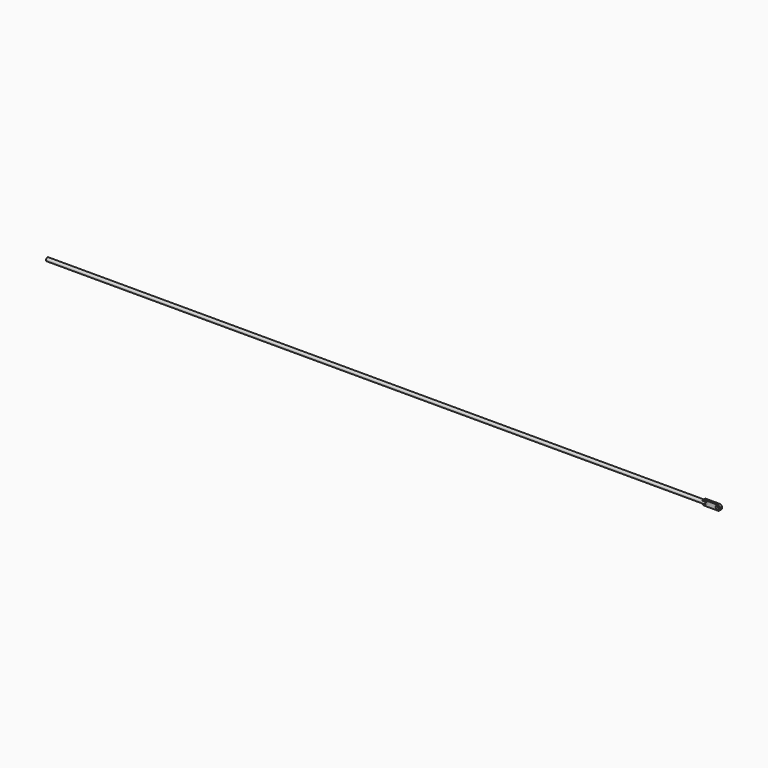
from build123d import *

# Parameters (mm, degrees)
F0_R         = 1.5875
F1_DEPTH     = 304.8
F3_DEPTH     = 1.0795
F4_T4_DEPTH  = 15.027948453
F4_S5_R      = 1.5875
F4_T6_DEPTH  = 9
F4_T10_DEPTH = 15.027948453
F4_S11_R     = 1.5875
F4_T12_DEPTH = 9
F5_R         = 1.5875
F6_DEPTH     = 2.6680001


# Not quite as in the source:
# - a fillet or chamfer that OpenCascade refuses, or shapes differently, is made with other operations: its cross-section is extruded or revolved along the edge and cut away or added


with BuildPart() as f1:
    # F0 (on Right) → F1 (new body, symmetric)
    with BuildSketch(Plane.YZ):
        Circle(F0_R)
    extrude(amount=F1_DEPTH, both=True)

    # F2 (on Front) → F3 (join, symmetric)
    with BuildSketch(Plane.XZ):
        with BuildLine():
            Line((304.7385620117, -2.3473887456), (317.4385620117, -2.3473887456))
            ThreePointArc((317.4385620117, -2.3473887456), (318.7856004299, -1.7894271638), (319.3435620117, -0.4423887456))
            Line((319.3435620117, -0.4423887456), (319.3435620117, 0.4423887456))
            ThreePointArc((319.3435620117, 0.4423887456), (318.7856004299, 1.7894271638), (317.4385620117, 2.3473887456))
            Line((317.4385620117, 2.3473887456), (304.7385620117, 2.3473887456))
            ThreePointArc((304.7385620117, 2.3473887456), (303.3915235936, 1.7894271638), (302.8335620117, 0.4423887456))
            Line((302.8335620117, 0.4423887456), (302.8335620117, -0.4423887456))
            ThreePointArc((302.8335620117, -0.4423887456), (303.3915235936, -1.7894271638), (304.7385620117, -2.3473887456))
        make_face()
    extrude(amount=F3_DEPTH, both=True)

    # F4: fillet of radius 2.54 on 2 edges, made by hand


with BuildPart() as f4_tool2:
    # F4_s3 → F4_t4 (new body)
    with BuildSketch(Plane.XY.offset(7.5139742265)):
        with BuildLine():
            ThreePointArc((307.34, -1.0795), (305.5439487758, -1.8234487758), (304.8, -3.6195))
            Line((304.8, -3.6195), (304.8, -1.0795))
            Line((304.8, -1.0795), (307.34, -1.0795))
        make_face()
    extrude(amount=-F4_T4_DEPTH)

    # F4_s5 → F4_t6 (intersect, symmetric)
    with BuildSketch(Plane.YZ.offset(306.1)):
        Circle(F4_S5_R)
    extrude(amount=F4_T6_DEPTH, both=True, mode=Mode.INTERSECT)


with BuildPart() as f1_1:
    add(f1.part)

    # F4_t1: union F4_tool2
    add(f4_tool2.part)


with BuildPart() as f4_tool8:
    # F4_s9 → F4_t10 (new body)
    with BuildSketch(Plane.XY.offset(7.5139742265)):
        with BuildLine():
            ThreePointArc((304.8, 3.6195), (305.5439487758, 1.8234487758), (307.34, 1.0795))
            Line((307.34, 1.0795), (304.8, 1.0795))
            Line((304.8, 1.0795), (304.8, 3.6195))
        make_face()
    extrude(amount=-F4_T10_DEPTH)

    # F4_s11 → F4_t12 (intersect, symmetric)
    with BuildSketch(Plane.YZ.offset(306.1)):
        Circle(F4_S11_R)
    extrude(amount=F4_T12_DEPTH, both=True, mode=Mode.INTERSECT)


with BuildPart() as f1_2:
    add(f1_1.part)

    # F4_t7: union F4_tool8
    add(f4_tool8.part)

    # F5 (on face) → F6 (cut, through all)
    with BuildSketch(Plane.XZ.offset(1.0795)):
        with Locations((316.8214559555, 0)):
            Circle(F5_R)
    extrude(amount=-F6_DEPTH, mode=Mode.SUBTRACT)


solid = f1_2.part
